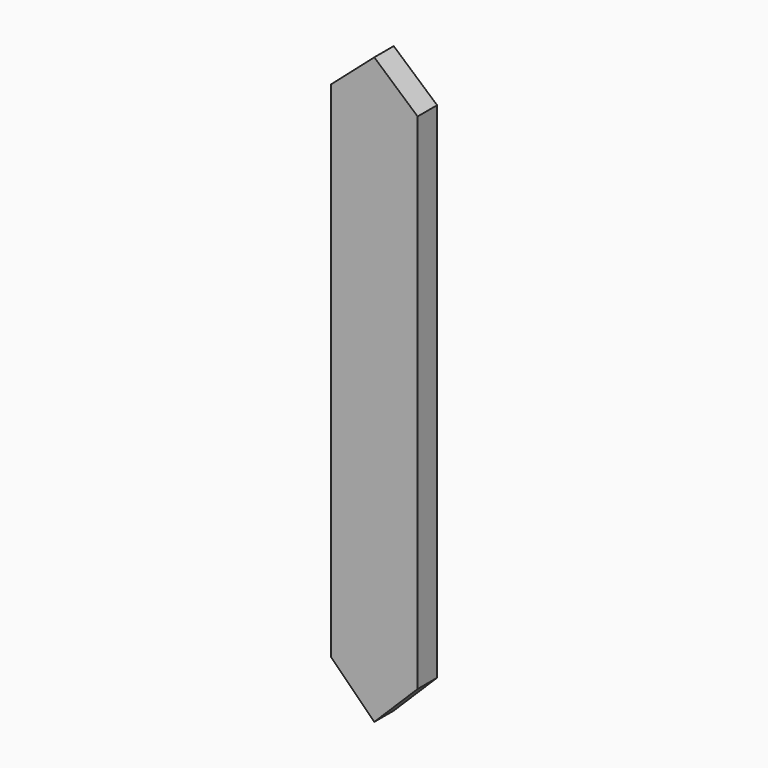
from build123d import *

# Parameters (mm, degrees)
F1_DEPTH = 5.08
F2_SIZE2 = 2.54
F2_SIZE  = 2.54
F3_W     = 296.9444543123
F3_H     = 473.9504568279
F4_DEPTH = 25.4
F5_DEPTH = 25.4


with BuildPart() as f1:
    # F0 (on Front) → F1 (new body, symmetric)
    with BuildSketch(Plane.XZ):
        with BuildLine():
            Line((-52.1713197231, 34.4429798424), (-58.770544827, 10.8928056434))
            add(Edge.make_bspline(
                [(-58.770544827, 10.8928056434), (-56.5008980701, 12.7169401311), (-52.1836149963, 16.1867774191), (-46.6481737875, 20.7689821181), (-42.103581434, 21.9474441882), (-37.1718262664, 20.3492743447), (-34.4780249811, 18.782172039), (-33.1500247121, 18.009616062)],
                knots=[0, 0, 0, 0, 0.243402605, 0.4629962541, 0.6364782013, 0.8207896592, 1, 1, 1, 1], degree=3))
            Line((-33.1500247121, 18.009616062), (0, 0))
            Line((0, 0), (33.1500247121, 18.009616062))
            add(Edge.make_bspline(
                [(58.770544827, 10.8928056434), (56.5008980701, 12.7169401311), (52.1836149963, 16.1867774191), (46.6481737875, 20.7689821181), (42.103581434, 21.9474441882), (37.1718262664, 20.3492743447), (34.4780249811, 18.782172039), (33.1500247121, 18.009616062)],
                knots=[0, 0, 0, 0, 0.243402605, 0.4629962541, 0.6364782013, 0.8207896592, 1, 1, 1, 1], degree=3))
            Line((58.770544827, 10.8928056434), (52.1713197231, 34.4429798424))
            add(Edge.make_bspline(
                [(52.1713197231, 34.4429798424), (50.9728401731, 36.5972375719), (48.6948112169, 40.6919770164), (44.4995729387, 45.251524036), (40.7511119594, 46.0496576718), (38.4311188014, 45.2100224851), (37.2595414519, 44.7860136628)],
                knots=[0, 0, 0, 0, 0.3036076859, 0.5770871099, 0.7864324897, 1, 1, 1, 1], degree=3))
            Line((37.2595414519, 44.7860136628), (12.3838605359, 31.5890572965))
            add(Edge.make_bspline(
                [(12.3838605359, 31.5890572965), (12.0116389407, 36.4336241706), (11.2801299785, 45.9544153649), (11.9072727509, 59.0755429111), (13.0446244948, 72.3270750889), (15.0430309606, 81.3553880474), (20.0484846376, 98.9141245501), (23.1138356658, 110.0238526226), (25.6900193935, 114.2539658888), (26.796290651, 116.070471704)],
                knots=[0, 0, 0, 0, 0.1554376564, 0.3054740514, 0.451951706, 0.5786332255, 0.7535204728, 0.8941561452, 1, 1, 1, 1], degree=3))
            add(Edge.make_bspline(
                [(26.796290651, 116.070471704), (27.3208616845, 122.376340647), (28.4465148418, 135.9078184294), (30.7430371303, 162.2435359747), (32.8128164069, 193.0751698329), (36.1980689164, 226.214181027), (36.6885878869, 228.6104286649), (36.1789175706, 231.6056884809), (34.578084839, 241.1608396791), (32.1815946616, 268.5632469899), (29.2022062034, 298.3654205907), (26.6745591694, 323.5321383941), (26.2740528758, 332.6532529053), (26.1084791273, 336.424022913)],
                knots=[0, 0, 0, 0, 0.0954552012, 0.2048329812, 0.3319664827, 0.4522041038, 0.4827906265, 0.5164846256, 0.5812786199, 0.6946646008, 0.8165569483, 0.9241626057, 1, 1, 1, 1], degree=3))
            Line((26.1084791273, 336.424022913), (0, 384.5021128654))
            Line((0, 384.5021128654), (-26.1084791273, 336.424022913))
            add(Edge.make_bspline(
                [(-26.796290651, 116.070471704), (-27.3208616845, 122.376340647), (-28.4465148418, 135.9078184294), (-30.7430371303, 162.2435359747), (-32.8128164069, 193.0751698329), (-36.1980689164, 226.214181027), (-36.6885878869, 228.6104286649), (-36.1789175706, 231.6056884809), (-34.578084839, 241.1608396791), (-32.1815946616, 268.5632469899), (-29.2022062034, 298.3654205907), (-26.6745591694, 323.5321383941), (-26.2740528758, 332.6532529053), (-26.1084791273, 336.424022913)],
                knots=[0, 0, 0, 0, 0.0954552012, 0.2048329812, 0.3319664827, 0.4522041038, 0.4827906265, 0.5164846256, 0.5812786199, 0.6946646008, 0.8165569483, 0.9241626057, 1, 1, 1, 1], degree=3))
            add(Edge.make_bspline(
                [(-12.3838605359, 31.5890572965), (-12.0116389407, 36.4336241706), (-11.2801299785, 45.9544153649), (-11.9072727509, 59.0755429111), (-13.0446244948, 72.3270750889), (-15.0430309606, 81.3553880474), (-20.0484846376, 98.9141245501), (-23.1138356658, 110.0238526226), (-25.6900193935, 114.2539658888), (-26.796290651, 116.070471704)],
                knots=[0, 0, 0, 0, 0.1554376564, 0.3054740514, 0.451951706, 0.5786332255, 0.7535204728, 0.8941561452, 1, 1, 1, 1], degree=3))
            Line((-12.3838605359, 31.5890572965), (-37.2595414519, 44.7860136628))
            add(Edge.make_bspline(
                [(-52.1713197231, 34.4429798424), (-50.9728401731, 36.5972375719), (-48.6948112169, 40.6919770164), (-44.4995729387, 45.251524036), (-40.7511119594, 46.0496576718), (-38.4311188014, 45.2100224851), (-37.2595414519, 44.7860136628)],
                knots=[0, 0, 0, 0, 0.3036076859, 0.5770871099, 0.7864324897, 1, 1, 1, 1], degree=3))
        make_face()
    extrude(amount=F1_DEPTH, both=True)

    # F2
    f2_edges = [f1.edges().sort_by_distance(p)[0] for p in [
        (-36.32486, 5.08, 226.315561),
        (-13.693841, 5.08, 74.863456),
        (-24.821701, 5.08, 38.187535),
        (-46.502615, 5.08, 42.946726),
        (-55.470932, 5.08, 22.667893),
        (-47.034517, 5.08, 20.082213),
        (-16.575012, 5.08, 9.004808),
        (16.575012, 5.08, 9.004808),
        (47.034517, 5.08, 20.082213),
        (55.470932, 5.08, 22.667893),
        (46.502615, 5.08, 42.946726),
        (24.821701, 5.08, 38.187535),
        (13.693841, 5.08, 74.863456),
        (36.32486, 5.08, 226.315561),
        (13.05424, 5.08, 360.463068),
        (-13.05424, 5.08, 360.463068),
        (-36.32486, -5.08, 226.315561),
        (-13.693841, -5.08, 74.863456),
        (-24.821701, -5.08, 38.187535),
        (-46.502615, -5.08, 42.946726),
        (-55.470932, -5.08, 22.667893),
        (-47.034517, -5.08, 20.082213),
        (-16.575012, -5.08, 9.004808),
        (16.575012, -5.08, 9.004808),
        (47.034517, -5.08, 20.082213),
        (55.470932, -5.08, 22.667893),
        (46.502615, -5.08, 42.946726),
        (24.821701, -5.08, 38.187535),
        (13.693841, -5.08, 74.863456),
        (36.32486, -5.08, 226.315561),
        (13.05424, -5.08, 360.463068),
        (-13.05424, -5.08, 360.463068),
    ]]
    chamfer(f2_edges, length=F2_SIZE, length2=F2_SIZE2)

    # F3 (on Front) → F4 (cut)
    with BuildSketch(Plane.XZ):
        with Locations((-3.1622722745, 199.3846241385)):
            Rectangle(F3_W, F3_H)
        Polygon((18.1035045534, 120.6582784653), (0, 102.6714965701), (-18.1035045534, 120.6582784653), (-18.1035045534, 331.0994207859), (0, 346.9451367855), (18.1035045534, 331.0994207859), align=None, mode=Mode.SUBTRACT)
    extrude(amount=-F4_DEPTH, mode=Mode.SUBTRACT)

    # F5 (cut): a face of the model
    f5_faces = [f1.faces().sort_by_distance(p)[0] for p in [
        (-9.5209365747, 0, 358.5443317782),
    ]]
    extrude(f5_faces, amount=-F5_DEPTH, mode=Mode.SUBTRACT)


solid = f1.part
